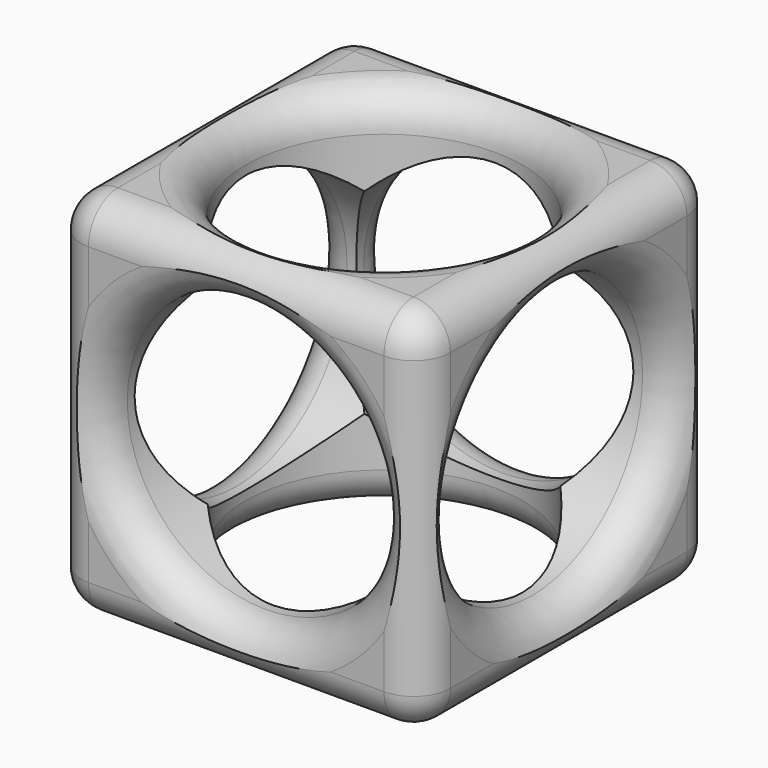
from build123d import *

# Parameters (mm, degrees)
F0_W         = 50.8
F0_H         = 50.8
F1_DEPTH     = 50.8
F2_R         = 19.05
F3_DEPTH     = 50.801
F4_R         = 19.05
F5_DEPTH     = 50.801
F6_R         = 19.05
F7_DEPTH     = 50.801
F8_T1_DEPTH  = 40.64
F8_T3_DEPTH  = 40.64
F8_T5_DEPTH  = 40.64
F8_S9_W      = 5.08
F8_S9_H      = 5.08
F8_T10_DEPTH = 5.08
F8_S15_W     = 5.08
F8_S15_H     = 5.08
F8_T16_DEPTH = 5.08
F8_S21_W     = 5.08
F8_S21_H     = 5.08
F8_T22_DEPTH = 5.08
F8_S27_W     = 5.08
F8_S27_H     = 5.08
F8_T28_DEPTH = 5.08
F8_S33_W     = 5.08
F8_S33_H     = 5.08
F8_T34_DEPTH = 5.08
F8_S39_W     = 5.08
F8_S39_H     = 5.08
F8_T40_DEPTH = 5.08
F8_S45_W     = 5.08
F8_S45_H     = 5.08
F8_T46_DEPTH = 5.08
F8_S51_W     = 5.08
F8_S51_H     = 5.08
F8_T52_DEPTH = 5.08


# Not quite as in the source:
# - a fillet or chamfer that OpenCascade refuses, or shapes differently, is made with other operations: its cross-section is extruded or revolved along the edge and cut away or added


with BuildPart() as f1:
    # F0 (on Front) → F1 (new body)
    with BuildSketch(Plane.XZ):
        with Locations((25.4, 25.4)):
            Rectangle(F0_W, F0_H)
    extrude(amount=F1_DEPTH)

    # F2 (on face) → F3 (cut, through all)
    with BuildSketch(Plane.XZ.offset(50.8)):
        with Locations((25.4, 25.4)):
            Circle(F2_R)
    extrude(amount=-F3_DEPTH, mode=Mode.SUBTRACT)

    # F4 (on face) → F5 (cut, through all)
    with BuildSketch(Plane.XY.offset(50.8)):
        with Locations((25.4, -25.4)):
            Circle(F4_R)
    extrude(amount=-F5_DEPTH, mode=Mode.SUBTRACT)

    # F6 (on face) → F7 (cut, through all)
    with BuildSketch(Plane(origin=(0, 0, 0), x_dir=(0, -1, 0), z_dir=(-1, 0, 0))):
        with Locations((25.4, 25.4)):
            Circle(F6_R)
    extrude(amount=-F7_DEPTH, mode=Mode.SUBTRACT)

    # F8: fillet of radius 5.08 on 18 edges, made by hand

    # F8_s2 → F8_t1 (cut)
    with BuildSketch(Plane.XZ.offset(5.08)):
        with BuildLine():
            ThreePointArc((0, 45.72), (1.4878975516, 49.3121024484), (5.08, 50.8))
            Line((5.08, 50.8), (0, 50.8))
            Line((0, 50.8), (0, 45.72))
        make_face()
        with BuildLine():
            ThreePointArc((0, 5.08), (1.4878975516, 1.4878975516), (5.08, 0))
            Line((5.08, 0), (0, 0))
            Line((0, 0), (0, 5.08))
        make_face()
        with BuildLine():
            ThreePointArc((45.72, 0), (49.3121024484, 1.4878975516), (50.8, 5.08))
            Line((50.8, 5.08), (50.8, 0))
            Line((50.8, 0), (45.72, 0))
        make_face()
        with BuildLine():
            ThreePointArc((45.72, 50.8), (49.3121024484, 49.3121024484), (50.8, 45.72))
            Line((50.8, 45.72), (50.8, 50.8))
            Line((50.8, 50.8), (45.72, 50.8))
        make_face()
    extrude(amount=F8_T1_DEPTH, mode=Mode.SUBTRACT)

    # F8_s4 → F8_t3 (cut)
    with BuildSketch(Plane.XY.offset(5.08)):
        with BuildLine():
            ThreePointArc((0, -5.08), (1.4878975516, -1.4878975516), (5.08, 0))
            Line((5.08, 0), (0, 0))
            Line((0, 0), (0, -5.08))
        make_face()
        with BuildLine():
            ThreePointArc((0, -45.72), (1.4878975516, -49.3121024484), (5.08, -50.8))
            Line((5.08, -50.8), (0, -50.8))
            Line((0, -50.8), (0, -45.72))
        make_face()
        with BuildLine():
            ThreePointArc((45.72, 0), (49.3121024484, -1.4878975516), (50.8, -5.08))
            Line((50.8, -5.08), (50.8, 0))
            Line((50.8, 0), (45.72, 0))
        make_face()
        with BuildLine():
            ThreePointArc((45.72, -50.8), (49.3121024484, -49.3121024484), (50.8, -45.72))
            Line((50.8, -45.72), (50.8, -50.8))
            Line((50.8, -50.8), (45.72, -50.8))
        make_face()
    extrude(amount=F8_T3_DEPTH, mode=Mode.SUBTRACT)

    # F8_s6 → F8_t5 (cut)
    with BuildSketch(Plane.YZ.offset(5.08)):
        with BuildLine():
            ThreePointArc((-5.08, 50.8), (-1.4878975516, 49.3121024484), (0, 45.72))
            Line((0, 45.72), (0, 50.8))
            Line((0, 50.8), (-5.08, 50.8))
        make_face()
        with BuildLine():
            ThreePointArc((0, 5.08), (-1.4878975516, 1.4878975516), (-5.08, 0))
            Line((-5.08, 0), (0, 0))
            Line((0, 0), (0, 5.08))
        make_face()
        with BuildLine():
            ThreePointArc((-45.72, 50.8), (-49.3121024484, 49.3121024484), (-50.8, 45.72))
            Line((-50.8, 45.72), (-50.8, 50.8))
            Line((-50.8, 50.8), (-45.72, 50.8))
        make_face()
        with BuildLine():
            ThreePointArc((-50.8, 5.08), (-49.3121024484, 1.4878975516), (-45.72, 0))
            Line((-45.72, 0), (-50.8, 0))
            Line((-50.8, 0), (-50.8, 5.08))
        make_face()
    extrude(amount=F8_T5_DEPTH, mode=Mode.SUBTRACT)


with BuildPart() as f8_tool8:
    # F8_s9 → F8_t10 (new body)
    with BuildSketch(Plane.YZ.offset(5.08)):
        with Locations((-2.54, 48.26)):
            Rectangle(F8_S9_W, F8_S9_H)
    extrude(amount=-F8_T10_DEPTH)

    # F8_s11 → F8_t12 (revolve, cut)
    with BuildSketch(Plane(origin=(5.08, -5.08, 45.72), x_dir=(0, -0.7071067812, -0.7071067812), z_dir=(0, 0.7071067812, -0.7071067812))):
        with BuildLine():
            ThreePointArc((0, -5.08), (5.08, 0), (0, 5.08))
            Line((0, 5.08), (0, -5.08))
        make_face()
    revolve(axis=Axis((5.08, -5.08, 45.72), (-1, 0, 0)), mode=Mode.SUBTRACT)


with BuildPart() as f1_1:
    add(f1.part)

    # F8_t7: cut F8_tool8
    add(f8_tool8.part, mode=Mode.SUBTRACT)


with BuildPart() as f8_tool14:
    # F8_s15 → F8_t16 (new body)
    with BuildSketch(Plane.YZ.offset(5.08)):
        with Locations((-48.26, 48.26)):
            Rectangle(F8_S15_W, F8_S15_H)
    extrude(amount=-F8_T16_DEPTH)

    # F8_s17 → F8_t18 (revolve, cut)
    with BuildSketch(Plane(origin=(5.08, -45.72, 45.72), x_dir=(0, 0.7071067812, -0.7071067812), z_dir=(0, 0.7071067812, 0.7071067812))):
        with BuildLine():
            ThreePointArc((0, -5.08), (5.08, 0), (0, 5.08))
            Line((0, 5.08), (0, -5.08))
        make_face()
    revolve(axis=Axis((5.08, -45.72, 45.72), (-1, 0, 0)), mode=Mode.SUBTRACT)


with BuildPart() as f1_2:
    add(f1_1.part)

    # F8_t13: cut F8_tool14
    add(f8_tool14.part, mode=Mode.SUBTRACT)


with BuildPart() as f8_tool20:
    # F8_s21 → F8_t22 (new body)
    with BuildSketch(Plane.YZ.offset(5.08)):
        with Locations((-2.54, 2.54)):
            Rectangle(F8_S21_W, F8_S21_H)
    extrude(amount=-F8_T22_DEPTH)

    # F8_s23 → F8_t24 (revolve, cut)
    with BuildSketch(Plane(origin=(5.08, -5.08, 5.08), x_dir=(0, -0.7071067812, 0.7071067812), z_dir=(0, -0.7071067812, -0.7071067812))):
        with BuildLine():
            ThreePointArc((0, -5.08), (5.08, 0), (0, 5.08))
            Line((0, 5.08), (0, -5.08))
        make_face()
    revolve(axis=Axis((5.08, -5.08, 5.08), (-1, 0, 0)), mode=Mode.SUBTRACT)


with BuildPart() as f1_3:
    add(f1_2.part)

    # F8_t19: cut F8_tool20
    add(f8_tool20.part, mode=Mode.SUBTRACT)


with BuildPart() as f8_tool26:
    # F8_s27 → F8_t28 (new body)
    with BuildSketch(Plane.YZ.offset(5.08)):
        with Locations((-48.26, 2.54)):
            Rectangle(F8_S27_W, F8_S27_H)
    extrude(amount=-F8_T28_DEPTH)

    # F8_s29 → F8_t30 (revolve, cut)
    with BuildSketch(Plane(origin=(5.08, -45.72, 5.08), x_dir=(0, 0.7071067812, 0.7071067812), z_dir=(0, -0.7071067812, 0.7071067812))):
        with BuildLine():
            ThreePointArc((0, -5.08), (5.08, 0), (0, 5.08))
            Line((0, 5.08), (0, -5.08))
        make_face()
    revolve(axis=Axis((5.08, -45.72, 5.08), (-1, 0, 0)), mode=Mode.SUBTRACT)


with BuildPart() as f1_4:
    add(f1_3.part)

    # F8_t25: cut F8_tool26
    add(f8_tool26.part, mode=Mode.SUBTRACT)


with BuildPart() as f8_tool32:
    # F8_s33 → F8_t34 (new body)
    with BuildSketch(Plane.XY.offset(45.72)):
        with Locations((48.26, -2.54)):
            Rectangle(F8_S33_W, F8_S33_H)
    extrude(amount=F8_T34_DEPTH)

    # F8_s35 → F8_t36 (revolve, cut)
    with BuildSketch(Plane(origin=(45.72, -5.08, 45.72), x_dir=(-0.7071067812, -0.7071067812, 0), z_dir=(-0.7071067812, 0.7071067812, 0))):
        with BuildLine():
            ThreePointArc((0, -5.08), (5.08, 0), (0, 5.08))
            Line((0, 5.08), (0, -5.08))
        make_face()
    revolve(axis=Axis((45.72, -5.08, 45.72), (0, 0, 1)), mode=Mode.SUBTRACT)


with BuildPart() as f1_5:
    add(f1_4.part)

    # F8_t31: cut F8_tool32
    add(f8_tool32.part, mode=Mode.SUBTRACT)


with BuildPart() as f8_tool38:
    # F8_s39 → F8_t40 (new body)
    with BuildSketch(Plane.XZ.offset(5.08)):
        with Locations((48.26, 2.54)):
            Rectangle(F8_S39_W, F8_S39_H)
    extrude(amount=-F8_T40_DEPTH)

    # F8_s41 → F8_t42 (revolve, cut)
    with BuildSketch(Plane(origin=(45.72, -5.08, 5.08), x_dir=(-0.7071067812, 0, 0.7071067812), z_dir=(-0.7071067812, 0, -0.7071067812))):
        with BuildLine():
            ThreePointArc((0, -5.08), (5.08, 0), (0, 5.08))
            Line((0, 5.08), (0, -5.08))
        make_face()
    revolve(axis=Axis((45.72, -5.08, 5.08), (0, 1, 0)), mode=Mode.SUBTRACT)


with BuildPart() as f1_6:
    add(f1_5.part)

    # F8_t37: cut F8_tool38
    add(f8_tool38.part, mode=Mode.SUBTRACT)


with BuildPart() as f8_tool44:
    # F8_s45 → F8_t46 (new body)
    with BuildSketch(Plane.XZ.offset(45.72)):
        with Locations((48.26, 2.54)):
            Rectangle(F8_S45_W, F8_S45_H)
    extrude(amount=F8_T46_DEPTH)

    # F8_s47 → F8_t48 (revolve, cut)
    with BuildSketch(Plane(origin=(45.72, -45.72, 5.08), x_dir=(-0.7071067812, 0, 0.7071067812), z_dir=(0.7071067812, 0, 0.7071067812))):
        with BuildLine():
            ThreePointArc((0, -5.08), (5.08, 0), (0, 5.08))
            Line((0, 5.08), (0, -5.08))
        make_face()
    revolve(axis=Axis((45.72, -45.72, 5.08), (0, -1, 0)), mode=Mode.SUBTRACT)


with BuildPart() as f1_7:
    add(f1_6.part)

    # F8_t43: cut F8_tool44
    add(f8_tool44.part, mode=Mode.SUBTRACT)


with BuildPart() as f8_tool50:
    # F8_s51 → F8_t52 (new body)
    with BuildSketch(Plane.XY.offset(45.72)):
        with Locations((48.26, -48.26)):
            Rectangle(F8_S51_W, F8_S51_H)
    extrude(amount=F8_T52_DEPTH)

    # F8_s53 → F8_t54 (revolve, cut)
    with BuildSketch(Plane(origin=(45.72, -45.72, 45.72), x_dir=(-0.7071067812, 0.7071067812, 0), z_dir=(0.7071067812, 0.7071067812, 0))):
        with BuildLine():
            ThreePointArc((0, -5.08), (5.08, 0), (0, 5.08))
            Line((0, 5.08), (0, -5.08))
        make_face()
    revolve(axis=Axis((45.72, -45.72, 45.72), (0, 0, 1)), mode=Mode.SUBTRACT)


with BuildPart() as f1_8:
    add(f1_7.part)

    # F8_t49: cut F8_tool50
    add(f8_tool50.part, mode=Mode.SUBTRACT)

    # F8_s55 → F8_t56 (revolve, cut)
    with BuildSketch(Plane.XY.offset(25.4)):
        with BuildLine():
            ThreePointArc((0, -49.53), (1.4878975516, -45.9378975516), (5.08, -44.45))
            Line((5.08, -44.45), (0, -44.45))
            Line((0, -44.45), (0, -49.53))
        make_face()
    revolve(axis=Axis((0, -25.4, 25.4), (-1, 0, 0)), mode=Mode.SUBTRACT)

    # F8_s57 → F8_t58 (revolve, cut)
    with BuildSketch(Plane.XY.offset(25.4)):
        with BuildLine():
            ThreePointArc((49.53, 0), (45.9378975516, -1.4878975516), (44.45, -5.08))
            Line((44.45, -5.08), (44.45, 0))
            Line((44.45, 0), (49.53, 0))
        make_face()
    revolve(axis=Axis((25.4, 0, 25.4), (0, -1, 0)), mode=Mode.SUBTRACT)

    # F8_s59 → F8_t60 (revolve, cut)
    with BuildSketch(Plane.XY.offset(25.4)):
        with BuildLine():
            ThreePointArc((50.8, -49.53), (49.3121024484, -45.9378975516), (45.72, -44.45))
            Line((45.72, -44.45), (50.8, -44.45))
            Line((50.8, -44.45), (50.8, -49.53))
        make_face()
    revolve(axis=Axis((50.8, -25.4, 25.4), (-1, 0, 0)), mode=Mode.SUBTRACT)

    # F8_s61 → F8_t62 (revolve, cut)
    with BuildSketch(Plane.XY.offset(25.4)):
        with BuildLine():
            ThreePointArc((49.53, -50.8), (45.9378975516, -49.3121024484), (44.45, -45.72))
            Line((44.45, -45.72), (44.45, -50.8))
            Line((44.45, -50.8), (49.53, -50.8))
        make_face()
    revolve(axis=Axis((25.4, -50.8, 25.4), (0, -1, 0)), mode=Mode.SUBTRACT)

    # F8_s63 → F8_t64 (revolve, cut)
    with BuildSketch(Plane.XZ.offset(25.4)):
        with BuildLine():
            ThreePointArc((49.53, 0), (45.9378975516, 1.4878975516), (44.45, 5.08))
            Line((44.45, 5.08), (44.45, 0))
            Line((44.45, 0), (49.53, 0))
        make_face()
    revolve(axis=Axis((25.4, -25.4, 0), (0, 0, 1)), mode=Mode.SUBTRACT)

    # F8_s65 → F8_t66 (revolve, cut)
    with BuildSketch(Plane.XZ.offset(25.4)):
        with BuildLine():
            ThreePointArc((49.53, 50.8), (45.9378975516, 49.3121024484), (44.45, 45.72))
            Line((44.45, 45.72), (44.45, 50.8))
            Line((44.45, 50.8), (49.53, 50.8))
        make_face()
    revolve(axis=Axis((25.4, -25.4, 50.8), (0, 0, 1)), mode=Mode.SUBTRACT)


solid = f1_8.part
